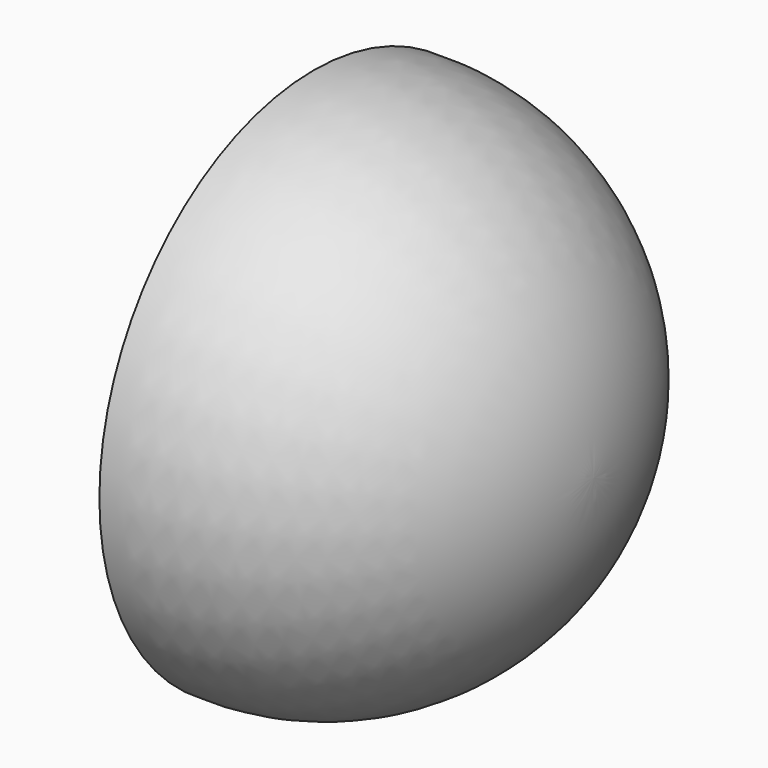
from build123d import *

# Parameters (mm, degrees)
F7_DEPTH  = 2.5
F13_DEPTH = 2
F49_DEPTH = 2


# Not quite as in the source:
# - ends of sketch curves that miss each other by under 0.0002 mm in the source are joined
# - the program builds the solid bodies; features that only make, move or delete a surface that nothing else refers to are left out


with BuildPart() as f1:
    # F0 (on Front) → F1 (revolve)
    with BuildSketch(Plane.XZ):
        with BuildLine():
            Line((0, 20), (0, 0))
            Line((0, 0), (20.9032140208, 0))
            ThreePointArc((20.9032140208, 0), (14.7145025663, 14.4554109076), (0, 20))
        make_face()
    revolve(axis=Axis((10.4516070104, 0, 0), (1, 0, 0)))

    # F2 (on Right) → F3 (revolve)
    with BuildSketch(Plane.YZ):
        with BuildLine():
            Line((-3, 0), (0, 0))
            Line((0, 0), (0, 3))
            ThreePointArc((0, 3), (-2.1378188048, 2.1378188048), (-3, 0))
        make_face()
    revolve(axis=Axis((0, -1.5, 0), (0, -1, 0)))

    # F4 (on face) → F5 (revolve)
    with BuildSketch(Plane(origin=(0, 0, 0), x_dir=(0, -1, 0), z_dir=(-1, 0, 0))):
        with BuildLine():
            Line((-3, 0), (0, 0))
            Line((0, 0), (0, 3))
            ThreePointArc((0, 3), (-2.1060516761, 2.1060516761), (-3, 0))
        make_face()
    revolve(axis=Axis((0, 1.5, 0), (0, 1, 0)))

    # F20 (on face) → F21 (revolve)
    with BuildSketch(Plane(origin=(0, 0, 0), x_dir=(0, -1, 0), z_dir=(-1, 0, 0))):
        with BuildLine():
            ThreePointArc((-7.6594431885, -3.8764923811), (-8.2749807984, -4.5285373926), (-7.6594431885, -5.1805824041))
            Line((-7.6594431885, -5.1805824041), (-7.6594431885, -3.8764923811))
        make_face()
    revolve(axis=Axis((0, 7.6594431885, -4.5285373926), (0, 0, 1)))

    # F22 (on face) → F23 (revolve)
    with BuildSketch(Plane(origin=(0, 0, 0), x_dir=(0, -1, 0), z_dir=(-1, 0, 0))):
        with BuildLine():
            ThreePointArc((12.7418441698, 5.2346289158), (12.1728994386, 4.6591833234), (12.7418441698, 4.083737731))
            Line((12.7418441698, 4.083737731), (12.7418441698, 5.2346289158))
        make_face()
    revolve(axis=Axis((0, -12.7418441698, 4.6591833234), (0, 0, 1)))

    # F24 (on face) → F25 (revolve)
    with BuildSketch(Plane(origin=(0, 0, 0), x_dir=(0, -1, 0), z_dir=(-1, 0, 0))):
        with BuildLine():
            ThreePointArc((-5.9676826932, -12.5175017115), (-6.7753176022, -13.3251366206), (-5.9676826932, -14.1327715296))
            Line((-5.9676826932, -14.1327715296), (-5.9676826932, -12.5175017115))
        make_face()
    revolve(axis=Axis((0, 5.9676826932, -13.3251366206), (0, 0, 1)))

    # F26 (on face) → F27 (revolve)
    with BuildSketch(Plane(origin=(0, 0, 0), x_dir=(0, -1, 0), z_dir=(-1, 0, 0))):
        with BuildLine():
            ThreePointArc((-2.6682941243, 17.2478277236), (-3.8004852056, 17.2364370857), (-3.7481172476, 16.1054003984))
            Line((-3.7481172476, 16.1054003984), (-2.6682941243, 17.2478277236))
        make_face()
    revolve(axis=Axis((0, 3.208205686, 16.676614061), (0, -0.6869139736, 0.7267387377)))

    # F30 (on face) → F31 (revolve)
    with BuildSketch(Plane(origin=(0, 0, 0), x_dir=(0, -1, 0), z_dir=(-1, 0, 0))):
        with BuildLine():
            ThreePointArc((2.065625973, 2.9552876949), (1.8622744828, 3.1655695777), (1.6589229926, 2.9552876949))
            Line((1.6589229926, 2.9552876949), (2.065625973, 2.9552876949))
        make_face()
    revolve(axis=Axis((0, -1.8622744828, 2.9552876949), (0, -1, 0)))

    # F32 (on face) → F33 (revolve)
    with BuildSketch(Plane(origin=(0, 0, 0), x_dir=(0, -1, 0), z_dir=(-1, 0, 0))):
        with BuildLine():
            ThreePointArc((4.7333193943, 2.0018331707), (4.6435543336, 2.0690382814), (4.5537892729, 2.0018331707))
            Line((4.5537892729, 2.0018331707), (4.7333193943, 2.0018331707))
        make_face()
    revolve(axis=Axis((0, -4.6435543336, 2.0018331707), (0, -1, 0)))

    # F34 (on face) → F35 (revolve)
    with BuildSketch(Plane(origin=(0, 0, 0), x_dir=(0, -1, 0), z_dir=(-1, 0, 0))):
        with BuildLine():
            Line((4.7080395743, -0.380108133), (4.4907717966, -0.380108133))
            ThreePointArc((4.4907717966, -0.380108133), (4.5994056854, -0.4801378843), (4.7080395743, -0.380108133))
        make_face()
    revolve(axis=Axis((0, -4.5994056854, -0.380108133), (0, -1, 0)))

    # F36 (on face) → F37 (revolve)
    with BuildSketch(Plane(origin=(0, 0, 0), x_dir=(0, -1, 0), z_dir=(-1, 0, 0))):
        with BuildLine():
            ThreePointArc((2.4876960088, -3.15255858), (2.3429562571, -2.9939137255), (2.1982165053, -3.15255858))
            Line((2.1982165053, -3.15255858), (2.4876960088, -3.15255858))
        make_face()
    revolve(axis=Axis((0, -2.3429562571, -3.15255858), (0, -1, 0)))

    # F38 (on face) → F39 (revolve)
    with BuildSketch(Plane(origin=(0, 0, 0), x_dir=(0, -1, 0), z_dir=(-1, 0, 0))):
        with BuildLine():
            ThreePointArc((3.7825170439, 0.9611435235), (3.6940083373, 1.0506368525), (3.6054996308, 0.9611435235))
            Line((3.6054996308, 0.9611435235), (3.7825170439, 0.9611435235))
        make_face()
    revolve(axis=Axis((0, -3.6940083373, 0.9611435235), (0, -1, 0)))

    # F40 (on face) → F41 (revolve)
    with BuildSketch(Plane(origin=(0, 0, 0), x_dir=(0, -1, 0), z_dir=(-1, 0, 0))):
        with BuildLine():
            ThreePointArc((0.5645051133, 3.9112772793), (0.4595427308, 4.0212758064), (0.3545803484, 3.9112772793))
            Line((0.3545803484, 3.9112772793), (0.5645051133, 3.9112772793))
        make_face()
    revolve(axis=Axis((0, -0.4595427308, 3.9112772793), (0, -1, 0)))

    # F42 (on face) → F43 (revolve)
    with BuildSketch(Plane(origin=(0, 0, 0), x_dir=(0, -1, 0), z_dir=(-1, 0, 0))):
        with BuildLine():
            ThreePointArc((5.4294881411, 0.7984926924), (5.4440247442, 1.0004788431), (5.2415728569, 1.005269587))
            Line((5.2415728569, 1.005269587), (5.4294881411, 0.7984926924))
        make_face()
    revolve(axis=Axis((0, -5.335530499, 0.9018811397), (0, -0.6725479403, -0.7400535575)))

    # F44 (on face) → F45 (revolve)
    with BuildSketch(Plane(origin=(0, 0, 0), x_dir=(0, -1, 0), z_dir=(-1, 0, 0))):
        with BuildLine():
            ThreePointArc((4.5250565745, -1.9389539957), (4.3312804717, -1.9511606938), (4.3379967101, -2.1452046931))
            Line((4.3379967101, -2.1452046931), (4.5250565745, -1.9389539957))
        make_face()
    revolve(axis=Axis((0, -4.4315266423, -2.0420793444), (0, -0.6718056347, 0.740727473)))

    # F46 (on face) → F47 (revolve)
    with BuildSketch(Plane(origin=(0, 0, 0), x_dir=(0, -1, 0), z_dir=(-1, 0, 0))):
        with BuildLine():
            Line((3.5201823339, -1.579977572), (3.3489386551, -1.579977572))
            ThreePointArc((3.3489386551, -1.579977572), (3.4345604945, -1.668621835), (3.5201823339, -1.579977572))
        make_face()
    revolve(axis=Axis((0, -3.4345604945, -1.579977572), (0, -1, 0)))


with BuildPart() as f7:
    # F6 (on face) → F7 (new body)
    with BuildSketch(Plane(origin=(0, 0, 0), x_dir=(0, -1, 0), z_dir=(-1, 0, 0))):
        with BuildLine():
            add(Edge.make_bspline(
                [(13.0212418735, -3.58440727), (10.7913677509, -1.6396786361), (6.5594301058, -8.7429022088), (2.3274924606, -15.8461257815), (8.7893042283, -10.6876308427), (15.2511159961, -5.5291359038), (13.0212418735, -3.58440727)],
                knots=[0, 0, 0, 2.0943951024, 2.0943951024, 4.1887902048, 4.1887902048, 6.2831853072, 6.2831853072, 6.2831853072], degree=2, weights=[1, 0.5, 1, 0.5, 1, 0.5, 1]))
        make_face()
    extrude(amount=F7_DEPTH)


with BuildPart() as f13:
    # F12 (on face) → F13 (new body)
    with BuildSketch(Plane(origin=(0, 0, 0), x_dir=(0, -1, 0), z_dir=(-1, 0, 0))):
        with BuildLine():
            add(Edge.make_bspline(
                [(10.9271379188, 7.5598936528), (12.4094731309, 10.030454188), (5.7548497871, 12.3432447088), (-0.8997735567, 14.6560352296), (4.2725145749, 9.8726841736), (9.4448027066, 5.0893331176), (10.9271379188, 7.5598936528)],
                knots=[0, 0, 0, 2.0943951024, 2.0943951024, 4.1887902048, 4.1887902048, 6.2831853072, 6.2831853072, 6.2831853072], degree=2, weights=[1, 0.5, 1, 0.5, 1, 0.5, 1]))
        make_face()
    extrude(amount=F13_DEPTH)


with BuildPart() as f29:
    # F28 (on face) → F29 (revolve)
    with BuildSketch(Plane(origin=(0, 0, 0), x_dir=(0, -1, 0), z_dir=(-1, 0, 0))):
        with BuildLine():
            ThreePointArc((3.4040999599, 3.4889467061), (3.2618925907, 3.612536586), (3.1196852215, 3.4889467061))
            Line((3.1196852215, 3.4889467061), (3.4040999599, 3.4889467061))
        make_face()
    revolve(axis=Axis((0, -3.2618925907, 3.4889467061), (0, -1, 0)))


with BuildPart() as f49:
    # F48 (on face) → F49 (new body)
    with BuildSketch(Plane(origin=(0, 0, 0), x_dir=(0, -1, 0), z_dir=(-1, 0, 0))):
        with BuildLine():
            add(Edge.make_bspline(
                [(-12.8653030843, -4.054680001), (-15.7865357239, -4.054680001), (-14.3259194041, -9.1504866723), (-12.8653030843, -14.2462933436), (-11.4046867644, -9.1504866723), (-9.9440704446, -4.054680001), (-12.8653030843, -4.054680001)],
                knots=[0, 0, 0, 2.0943951024, 2.0943951024, 4.1887902048, 4.1887902048, 6.2831853072, 6.2831853072, 6.2831853072], degree=2, weights=[1, 0.5, 1, 0.5, 1, 0.5, 1]))
        make_face()
    extrude(amount=F49_DEPTH)


solid = Compound([f1.part, f7.part, f13.part, f29.part, f49.part])
